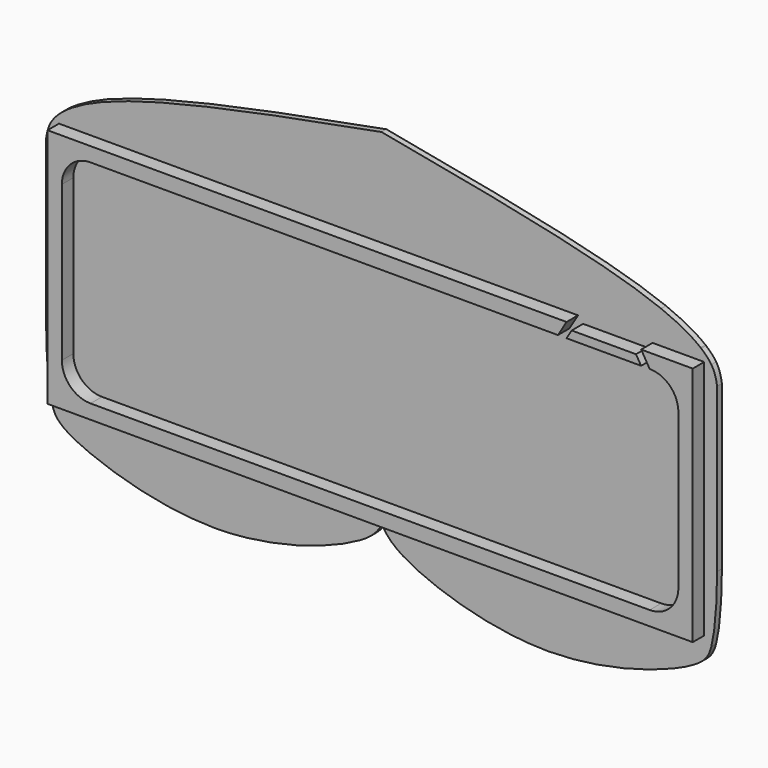
from build123d import *

# Parameters (mm, degrees)
F0_W     = 584.2
F0_H     = 219.71
F1_DEPTH = 5.334
F2_W     = 571.5
F2_H     = 213.36
F2_W_2   = 546.1
F2_H_2   = 187.96
F3_DEPTH = 12.7
F4_R     = 25.4
F6_DEPTH = 12.7
F8_DEPTH = 5.334


# Not quite as in the source:
# - a feature names something its author has since deleted; it is built from what else it names


with BuildPart() as f1:
    # F0 (on Front) → F1 (new body)
    with BuildSketch(Plane.XZ):
        with Locations((-292.1, 109.855)):
            Rectangle(F0_W, F0_H)
    extrude(amount=F1_DEPTH)

    # F2 (on face) → F3 (join)
    with BuildSketch(Plane.XZ.offset(5.334)):
        with Locations((-292.1, 113.03)):
            Rectangle(F2_W, F2_H)
        with Locations((-292.1, 113.03)):
            Rectangle(F2_W_2, F2_H_2, mode=Mode.SUBTRACT)
    extrude(amount=F3_DEPTH)

    # F4
    f4_edges = [f1.edges().sort_by_distance(p)[0] for p in [
        (-565.15, -11.684, 207.01),
        (-19.05, -11.684, 207.01),
        (-19.05, -11.684, 19.05),
        (-565.15, -11.684, 19.05),
    ]]
    fillet(f4_edges, radius=F4_R)

    # F5 (on face) → F6 (cut)
    with BuildSketch(Plane.XZ.offset(18.034)):
        Polygon((-118.11, 219.71), (-125.73, 207.01), (-118.11, 207.01), (-113.5820166854, 214.5566388576), (-110.49, 219.71), align=None)
        Polygon((-56.5979833146, 214.5566388576), (-52.07, 207.01), (-44.45, 207.01), (-52.07, 219.71), (-59.69, 219.71), align=None)
        Polygon((-59.69, 219.71), (-110.49, 219.71), (-113.5820166854, 214.5566388576), (-56.5979833146, 214.5566388576), align=None)
    extrude(amount=-F6_DEPTH, mode=Mode.SUBTRACT)

    # F7 (on face) → F8 (join)
    with BuildSketch(Plane(origin=(0, 0, 0), x_dir=(-1, 0, 0), z_dir=(0, 1, 0))):
        with BuildLine():
            Line((292.1, 0), (0, 0))
            add(Edge.make_bspline(
                [(13.97, -18.4182160117), (5.1776683434, -12.9300591082), (2.1993531585, -8.4306227348), (0, 0)],
                knots=[0.6884256157, 0.6884256157, 0.6884256157, 0.6884256157, 0.8055577438, 0.8055577438, 0.8055577438, 0.8055577438], degree=3))
            Line((13.97, -18.4182160117), (273.05, -18.4182160117))
            add(Edge.make_bspline(
                [(292.1, 0), (287.8348745006, -6.4171904537), (283.3704909948, -12.0241872437), (273.05, -18.4182160117)],
                knots=[0, 0, 0, 0, 0.1254053332, 0.1254053332, 0.1254053332, 0.1254053332], degree=3))
        make_face()
        with BuildLine():
            add(Edge.make_bspline(
                [(0, 0), (-3.4777348873, 13.330951736), (-5.0077822241, 36.49129499), (-5.08, 59.9872617497)],
                knots=[0.8055577438, 0.8055577438, 0.8055577438, 0.8055577438, 0.9907733318, 0.9907733318, 0.9907733318, 0.9907733318], degree=3))
            Line((0, 0), (0, 109.855))
            Line((0, 109.855), (-5.08, 109.855))
            Line((-5.08, 109.855), (-5.08, 63.5))
            Line((-5.08, 63.5), (-5.08, 59.9872617497))
        make_face()
        with BuildLine():
            Line((273.05, -18.4182160117), (13.97, -18.4182160117))
            add(Edge.make_bspline(
                [(143.51, -50.8), (89.8146392781, -50.5091658601), (35.101098408, -31.6082079428), (13.97, -18.4182160117)],
                knots=[0.4069154744, 0.4069154744, 0.4069154744, 0.4069154744, 0.6884256157, 0.6884256157, 0.6884256157, 0.6884256157], degree=3))
            Line((143.51, -50.8), (146.0426574413, -50.8))
            add(Edge.make_bspline(
                [(273.05, -18.4182160117), (250.2469136161, -32.545798741), (198.8550496381, -50.5155722463), (146.0426574413, -50.8)],
                knots=[0.1254053332, 0.1254053332, 0.1254053332, 0.1254053332, 0.4024879494, 0.4024879494, 0.4024879494, 0.4024879494], degree=3))
        make_face()
        with BuildLine():
            Line((584.2, 0), (292.1, 0))
            add(Edge.make_bspline(
                [(292.1, 0), (295.2511238563, -6.7739107165), (300.4280406329, -12.1526213408), (311.15, -18.4182160117)],
                knots=[0, 0, 0, 0, 0.1254053332, 0.1254053332, 0.1254053332, 0.1254053332], degree=3))
            Line((311.15, -18.4182160117), (570.23, -18.4182160117))
            add(Edge.make_bspline(
                [(570.23, -18.4182160117), (579.0383616328, -12.9277742975), (582.0053728244, -8.4368679309), (584.2, 0)],
                knots=[0.6884256157, 0.6884256157, 0.6884256157, 0.6884256157, 0.8055577438, 0.8055577438, 0.8055577438, 0.8055577438], degree=3))
        make_face()
        with BuildLine():
            Line((-5.08, 109.855), (0, 109.855))
            Line((0, 109.855), (0, 219.71))
            add(Edge.make_bspline(
                [(0, 219.71), (-3.3633398359, 214.4958413315), (-4.221669918, 209.4829206658), (-5.08, 204.47)],
                knots=[0.8528806378, 0.8528806378, 0.8528806378, 0.8528806378, 1, 1, 1, 1], degree=3))
            Line((-5.08, 204.47), (-5.08, 109.855))
        make_face()
        with BuildLine():
            Line((570.23, -18.4182160117), (311.15, -18.4182160117))
            add(Edge.make_bspline(
                [(311.15, -18.4182160117), (334.9383025593, -32.3193936455), (386.0216290424, -50.5861863086), (438.8223695347, -50.8)],
                knots=[0.1254053332, 0.1254053332, 0.1254053332, 0.1254053332, 0.4036361962, 0.4036361962, 0.4036361962, 0.4036361962], degree=3))
            Line((438.8223695347, -50.8), (440.69, -50.8))
            add(Edge.make_bspline(
                [(440.69, -50.8), (494.1504250391, -50.5826159423), (549.0603758608, -31.6136991551), (570.23, -18.4182160117)],
                knots=[0.4069154744, 0.4069154744, 0.4069154744, 0.4069154744, 0.6884256157, 0.6884256157, 0.6884256157, 0.6884256157], degree=3))
        make_face()
        with BuildLine():
            Line((584.2, 109.855), (584.2, 0))
            add(Edge.make_bspline(
                [(584.2, 0), (587.6660611317, 13.3246778013), (589.2055548561, 36.4918183962), (589.28, 59.9101174948)],
                knots=[0.8055577438, 0.8055577438, 0.8055577438, 0.8055577438, 0.9905491269, 0.9905491269, 0.9905491269, 0.9905491269], degree=3))
            Line((589.28, 59.9101174948), (589.28, 63.5))
            Line((589.28, 63.5), (589.28, 109.855))
            Line((589.28, 109.855), (584.2, 109.855))
        make_face()
        with BuildLine():
            add(Edge.make_bspline(
                [(8.9497229668, 229.3903513516), (5.0117556013, 226.1203537614), (2.0435071593, 222.8780326962), (0, 219.71)],
                knots=[0.7634934559, 0.7634934559, 0.7634934559, 0.7634934559, 0.8528806378, 0.8528806378, 0.8528806378, 0.8528806378], degree=3))
            Line((0, 219.71), (292.1, 219.71))
            Line((292.1, 219.71), (8.9497229668, 229.3903513516))
        make_face()
        with BuildLine():
            Line((584.2, 219.71), (584.2, 109.855))
            Line((584.2, 109.855), (589.28, 109.855))
            Line((589.28, 109.855), (589.28, 204.47))
            add(Edge.make_bspline(
                [(584.2, 219.71), (587.5633398359, 214.4958413315), (588.421669918, 209.4829206658), (589.28, 204.47)],
                knots=[0.8528806378, 0.8528806378, 0.8528806378, 0.8528806378, 1, 1, 1, 1], degree=3))
        make_face()
        with BuildLine():
            add(Edge.make_bspline(
                [(9.5340725562, 229.87), (9.3369695017, 229.7100546344), (9.1421880555, 229.5501699377), (8.9497229668, 229.3903513516)],
                knots=[0.759124727, 0.759124727, 0.759124727, 0.759124727, 0.7634934559, 0.7634934559, 0.7634934559, 0.7634934559], degree=3))
            Line((8.9497229668, 229.3903513516), (292.1, 219.71))
            Line((292.1, 219.71), (575.2502770332, 229.3903513516))
            add(Edge.make_bspline(
                [(574.6659274438, 229.87), (574.8630304983, 229.7100546344), (575.0578119445, 229.5501699377), (575.2502770332, 229.3903513516)],
                knots=[0.759124727, 0.759124727, 0.759124727, 0.759124727, 0.7634934559, 0.7634934559, 0.7634934559, 0.7634934559], degree=3))
            Line((574.6659274438, 229.87), (539.75, 229.87))
            Line((539.75, 229.87), (292.1, 229.87))
            Line((292.1, 229.87), (44.45, 229.87))
            Line((44.45, 229.87), (9.5340725562, 229.87))
        make_face()
        with BuildLine():
            Line((575.2502770332, 229.3903513516), (292.1, 219.71))
            Line((292.1, 219.71), (584.2, 219.71))
            add(Edge.make_bspline(
                [(575.2502770332, 229.3903513516), (579.1882443987, 226.1203537614), (582.1564928407, 222.8780326962), (584.2, 219.71)],
                knots=[0.7634934559, 0.7634934559, 0.7634934559, 0.7634934559, 0.8528806378, 0.8528806378, 0.8528806378, 0.8528806378], degree=3))
        make_face()
        with BuildLine():
            add(Edge.make_bspline(
                [(44.45, 248.92), (28.9100061464, 242.7028057711), (17.3818410687, 236.2383143168), (9.5340725562, 229.87)],
                knots=[0.5851813382, 0.5851813382, 0.5851813382, 0.5851813382, 0.759124727, 0.759124727, 0.759124727, 0.759124727], degree=3))
            Line((9.5340725562, 229.87), (44.45, 229.87))
            Line((44.45, 229.87), (44.45, 248.92))
        make_face()
        with BuildLine():
            Line((44.45, 248.92), (44.45, 229.87))
            Line((44.45, 229.87), (292.1, 229.87))
            Line((292.1, 229.87), (292.1, 306.07))
            add(Edge.make_bspline(
                [(292.1, 306.07), (194.4148678752, 287.9529601014), (96.7297357504, 269.8359202028), (44.45, 248.92)],
                knots=[0, 0, 0, 0, 0.5851813382, 0.5851813382, 0.5851813382, 0.5851813382], degree=3))
        make_face()
        with BuildLine():
            Line((539.75, 229.87), (574.6659274438, 229.87))
            add(Edge.make_bspline(
                [(539.75, 248.92), (555.2899938536, 242.7028057711), (566.8181589313, 236.2383143168), (574.6659274438, 229.87)],
                knots=[0.5851813382, 0.5851813382, 0.5851813382, 0.5851813382, 0.759124727, 0.759124727, 0.759124727, 0.759124727], degree=3))
            Line((539.75, 248.92), (539.75, 229.87))
        make_face()
        with BuildLine():
            Line((292.1, 306.07), (292.1, 229.87))
            Line((292.1, 229.87), (539.75, 229.87))
            Line((539.75, 229.87), (539.75, 248.92))
            add(Edge.make_bspline(
                [(292.1, 306.07), (389.7851321248, 287.9529601014), (487.4702642496, 269.8359202028), (539.75, 248.92)],
                knots=[0, 0, 0, 0, 0.5851813382, 0.5851813382, 0.5851813382, 0.5851813382], degree=3))
        make_face()
    extrude(amount=-F8_DEPTH)


solid = f1.part
